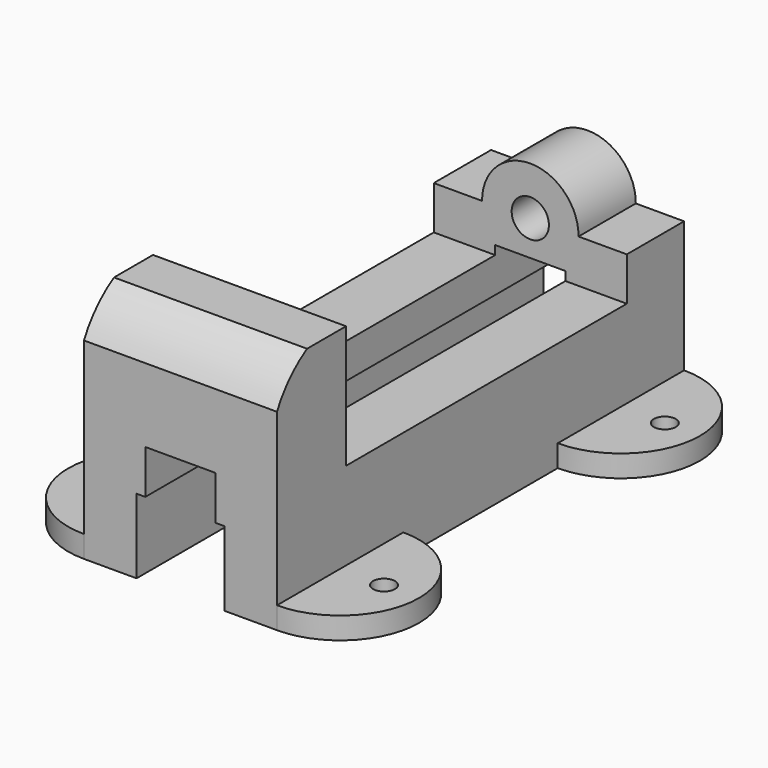
from build123d import *

# Parameters (mm, degrees)
F1_DEPTH = 2750
F2_R     = 1125
F2_R_2   = 156
F3_DEPTH = 312
F5_DEPTH = 9516.50351
F6_R     = 265.5
F7_DEPTH = 2759.03485


with BuildPart() as f1:
    # F0 (on Right) → F1 (new body)
    with BuildSketch(Plane.YZ):
        with BuildLine():
            Line((-2395, 1656), (-3089.0144090723, 1656))
            ThreePointArc((-3089.0144090723, 1656), (-3398.6783356879, 1408.816364228), (-3625, 1083.5933615001))
            Line((-3625, 1083.5933615001), (-3625, -1656))
            Line((-3625, -1656), (0, -1656))
            Line((0, -1656), (0, -94))
            Line((0, -94), (-2395, -94))
            Line((-2395, -94), (-2395, 1656))
        make_face()
        Polygon((2605, -94), (0, -94), (0, -1656), (3625, -1656), (3625, 1656), (2605, 1656), align=None)
    extrude(amount=F1_DEPTH)

    # F2 (on face) → F3 (join)
    with BuildSketch(Plane(origin=(0, 0, -1656), x_dir=(1, 0, 0), z_dir=(0, 0, -1))):
        with Locations((0, 2500)):
            Circle(F2_R)
        with Locations((-625, 2500)):
            Circle(F2_R_2, mode=Mode.SUBTRACT)
        with Locations((2750, 2500)):
            Circle(F2_R)
        with Locations((3375, 2500)):
            Circle(F2_R_2, mode=Mode.SUBTRACT)
        with Locations((2750, -2500)):
            Circle(F2_R)
        with Locations((3375, -2500)):
            Circle(F2_R_2, mode=Mode.SUBTRACT)
        with Locations((0, -2500)):
            Circle(F2_R)
        with Locations((-625, -2500)):
            Circle(F2_R_2, mode=Mode.SUBTRACT)
    extrude(amount=-F3_DEPTH)

    # F4 (on face) → F5 (cut)
    with BuildSketch(Plane.XZ.offset(3625)):
        Polygon((1375, 32), (875, 32), (875, -594), (750, -594), (750, -1656), (875, -1656), (1875, -1656), (2000, -1656), (2000, -594), (1875, -594), (1875, 32), align=None)
    extrude(amount=-F5_DEPTH, mode=Mode.SUBTRACT)

    # F6 (on face) → F7 (cut)
    with BuildSketch(Plane(origin=(0, 3625, 0), x_dir=(-1, 0, 0), z_dir=(0, 1, 0))):
        with Locations((-1375, 531)):
            Circle(F6_R)
        with BuildLine():
            ThreePointArc((-2061.9735275378, 524.9690413475), (-1375, 1218), (-688.0264724622, 524.9690413475))
            Line((-688.0264724622, 524.9690413475), (0, 524.9690413475))
            Line((0, 524.9690413475), (0, 1656))
            Line((0, 1656), (-2750, 1656))
            Line((-2750, 1656), (-2750, 524.9690413475))
            Line((-2750, 524.9690413475), (-2061.9735275378, 524.9690413475))
        make_face()
    extrude(amount=-F7_DEPTH, mode=Mode.SUBTRACT)


solid = f1.part
